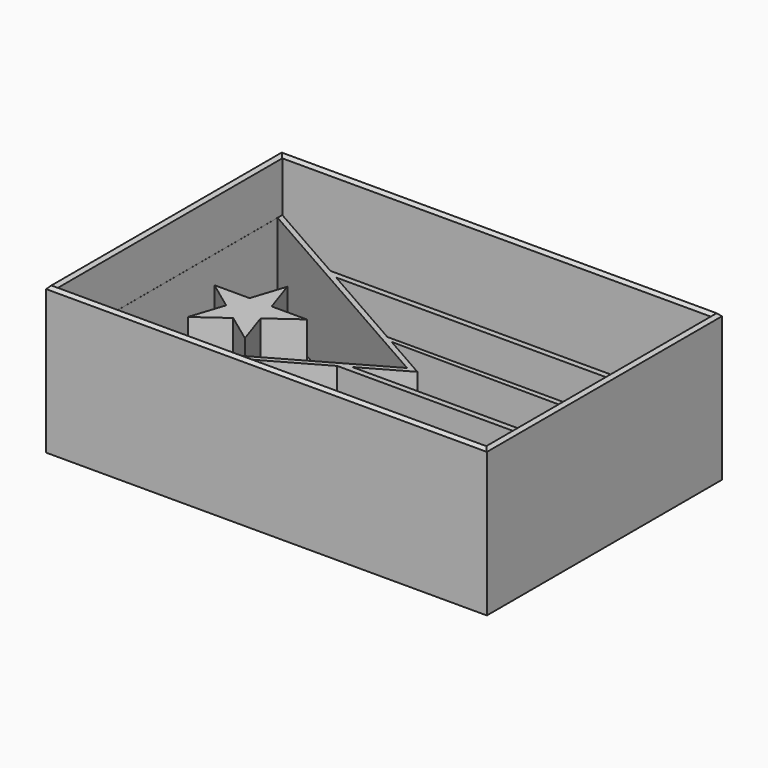
from build123d import *

# Parameters (mm, degrees)
F1_W      = 75
F1_H      = 49.9875
F2_DEPTH  = 25
F3_W      = 73
F3_H      = 47.9875
F4_DEPTH  = 25
F5_SIZE2  = 0.49999
F5_SIZE   = 0.49999
F7_DEPTH  = 16
F9_DEPTH  = 16
F11_DEPTH = 16
F13_DEPTH = 16
F15_DEPTH = 16
F17_DEPTH = 16
F19_DEPTH = 16
F21_DEPTH = 0.4
F23_DEPTH = 0.4
F25_DEPTH = 0.4


# Not quite as in the source:
# - a fillet or chamfer is up to 0.001 mm smaller than in the source, because OpenCascade refuses the exact size


with BuildPart() as f2:
    # F1 (on Top) → F2 (new body)
    with BuildSketch(Plane.XY):
        with Locations((-1.6757239815, -4.8845620042)):
            Rectangle(F1_W, F1_H)
    extrude(amount=F2_DEPTH)

    # F3 (on Top) → F4 (cut)
    with BuildSketch(Plane.XY):
        with Locations((-1.6757239815, -4.8845620042)):
            Rectangle(F3_W, F3_H)
    extrude(amount=F4_DEPTH, mode=Mode.SUBTRACT)

    # F5 (size 0.5 and 0.5 in the source; OpenCascade refuses exactly that, so slightly less here)
    f5_edges = [f2.edges().sort_by_distance(p)[0] for p in [
        (-1.675724, -29.878312, 25),
        (-39.175724, -4.884562, 25),
        (35.824276, -4.884562, 25),
        (-1.675724, 20.109188, 25),
        (-1.675724, -28.878312, 25),
        (34.824276, -4.884562, 25),
        (-1.675724, 19.109188, 25),
        (-38.175724, -4.884562, 25),
    ]]
    chamfer(f5_edges, length=F5_SIZE, length2=F5_SIZE2)

    # F6 (on Top) → F7 (join)
    with BuildSketch(Plane.XY):
        Polygon((4.0175896138, -4.9000722356), (-38.1757239815, 19.1091879958), (-38.1757239815, -28.8783120042), align=None)
    extrude(amount=F7_DEPTH)

    # F8 (on Top) → F9 (cut)
    with BuildSketch(Plane.XY):
        Polygon((2.2694178753, -4.8994258076), (-38.1653830409, 18.1091879958), (-38.1653830409, -27.8783120042), align=None)
    extrude(amount=F9_DEPTH, mode=Mode.SUBTRACT)

    # F10 (on Top) → F11 (join)
    with BuildSketch(Plane.XY):
        Polygon((34.8242760185, 10.5531314617), (-23.1395099124, 10.5531314617), (-21.3821332507, 9.5531314617), (34.8242760185, 9.5531314617), align=None)
    extrude(amount=F11_DEPTH)

    # F12 (on Top) → F13 (join)
    with BuildSketch(Plane.XY):
        Polygon((34.8242760185, 0.4371882224), (-5.3619873524, 0.4371882224), (-4.0423821136, -0.3137067153), (34.8242760185, -0.5628117776), align=None)
    extrude(amount=F13_DEPTH)

    # F14 (on Top) → F15 (join)
    with BuildSketch(Plane.XY):
        Polygon((34.8242760185, -9.2302871699), (-3.6020738153, -9.2302871699), (-5.3617239815, -10.2302871699), (34.8242760185, -10.2302871699), align=None)
    extrude(amount=F15_DEPTH)

    # F16 (on Top) → F17 (join)
    with BuildSketch(Plane.XY):
        Polygon((-21.6990868828, -19.5147251875), (-23.1394399608, -20.3332703197), (34.8242760185, -20.5147251875), (34.8242760185, -19.5147251875), align=None)
    extrude(amount=F17_DEPTH)

    # F22 (on Top) → F23 (join)
    with BuildSketch(Plane.XY):
        Polygon((28.8242760185, 19.1091879958), (14.8242760185, 19.1091879958), (14.8242760185, -29.8783120042), (28.8242760185, -29.8783120042), (28.8242760185, 4.2719491757), align=None)
    extrude(amount=F23_DEPTH)

    # F24 (on Top) → F25 (join)
    with BuildSketch(Plane.XY):
        Polygon((2.5, 19.1091879958), (-2.5, 19.1091879958), (-2.5, -28.8783120042), (2.5, -28.8783120042), (2.5, 7.0442273282), align=None)
    extrude(amount=F25_DEPTH)


with BuildPart() as f19:
    # F18 (on Top) → F19 (new body)
    with BuildSketch(Plane.XY):
        Polygon((-22.8562415051, -2.3057359916), (-24.7815981912, 3.4265754099), (-26.6346354038, -2.2761789151), (-32.6149091125, -2.2761789151), (-27.7723465115, -5.8351713233), (-29.6539459378, -11.6258263588), (-24.7676242143, -8.0960066989), (-19.9255160506, -11.6546651231), (-21.8570372557, -5.9040002689), (-16.8759677964, -2.3057359916), align=None)
    extrude(amount=F19_DEPTH)


with BuildPart() as f21:
    # F20 (on Top) → F21 (new body)
    with BuildSketch(Plane.XY):
        Polygon((-18.1757239815, 19.1091879958), (-32.1757239815, 19.1091879958), (-32.1757239815, 8.0351457), (-32.1757239815, -28.8783120042), (-18.1757239815, -28.8783120042), align=None)
    extrude(amount=F21_DEPTH)


solid = Compound([f2.part, f19.part, f21.part])
